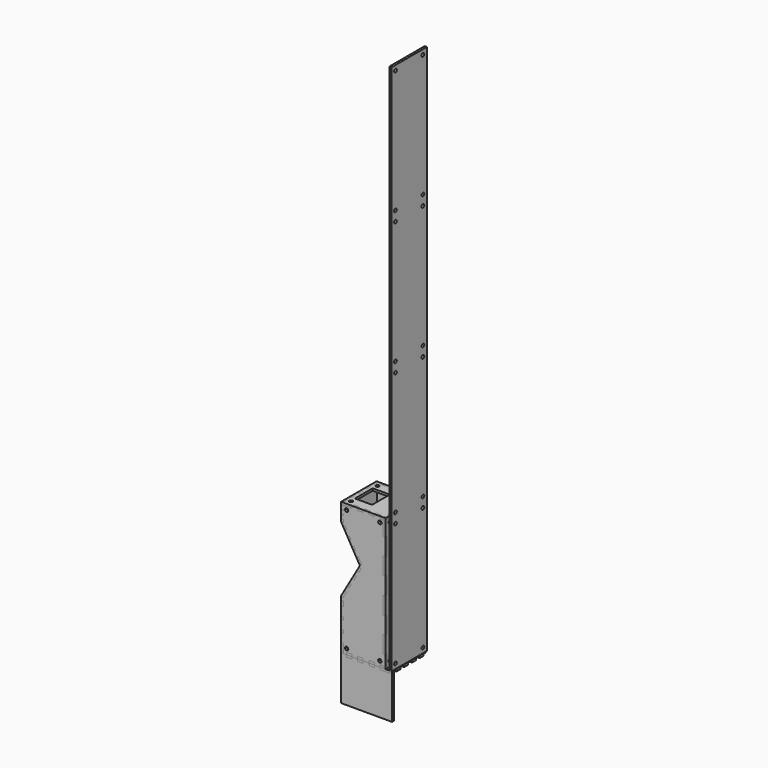
from build123d import *

# Parameters (mm, degrees)
F5_W      = 6
F5_H      = 4
F5_W_2    = 10
F5_W_3    = 4
F5_H_2    = 4.9052353799
F5_H_3    = 8.75
F5_R      = 3
F5_W_4    = 31
F5_H_4    = 40
F5_H_5    = 5.8447646201
F25_DEPTH = 4
F7_R      = 3
F7_W      = 4
F7_H      = 30
F7_H_2    = 31.25
F7_H_3    = 22.5
F26_DEPTH = 4
F3_R      = 3
F27_DEPTH = 4
F9_W      = 6
F9_H      = 4
F9_W_2    = 10
F9_R      = 3
F9_W_3    = 4
F9_H_2    = 14.5947646201
F9_H_3    = 8.75
F9_H_4    = 4.9052353799
F28_DEPTH = 4
F11_R     = 3
F29_DEPTH = 4
F30_DEPTH = 4
F31_DEPTH = 4
F32_DEPTH = 4
F33_DEPTH = 4
F34_DEPTH = 4
F35_DEPTH = 4
F36_DEPTH = 4
F37_DEPTH = 4
F38_DEPTH = 4
F19_R     = 25
F39_DEPTH = 4
F40_DEPTH = 4
F22_W     = 80
F22_H     = 240
F22_R     = 3
F41_DEPTH = 4
F24_R     = 3
F24_W     = 31
F24_H     = 40
F42_DEPTH = 4
F43_DEPTH = 4
F23_W     = 6
F23_H     = 4
F23_W_2   = 4
F23_H_2   = 8.75
F23_W_3   = 10
F23_H_3   = 4.9052353799
F44_DEPTH = 4
F23_H_4   = 5.8447646201
F45_DEPTH = 4


# Not quite as in the source:
# - a feature names something its author has since deleted; it is built from what else it names


with BuildPart() as f25:
    # F5 (on line) → F25 (new body)
    with BuildSketch(Plane.XY.offset(240)):
        with Locations((-73, 78)):
            Rectangle(F5_W, F5_H)
        with Locations((-55, 78)):
            Rectangle(F5_W_2, F5_H)
        with Locations((-35, 78)):
            Rectangle(F5_W_2, F5_H)
        with Locations((-15, 78)):
            Rectangle(F5_W_2, F5_H)
        with Locations((-2, 78)):
            Rectangle(F5_W_3, F5_H)
        with Locations((-2, 73.54738231)):
            Rectangle(F5_W_3, F5_H_2)
        with Locations((-2, 57.9697646201)):
            Rectangle(F5_W_3, F5_H_3)
        with Locations((-2, 40.4697646201)):
            Rectangle(F5_W_3, F5_H_3)
        with Locations((-2, 22.9697646201)):
            Rectangle(F5_W_3, F5_H_3)
        with Locations((-25, 2)):
            Rectangle(F5_W_2, F5_H)
        with Locations((-45, 2)):
            Rectangle(F5_W_2, F5_H)
        with Locations((-65, 2)):
            Rectangle(F5_W_2, F5_H)
        with Locations((-78, 66.7197646201)):
            Rectangle(F5_W_3, F5_H_3)
        with Locations((-78, 49.2197646201)):
            Rectangle(F5_W_3, F5_H_3)
        with Locations((-78, 31.7197646201)):
            Rectangle(F5_W_3, F5_H_3)
        with Locations((-78, 14.2197646201)):
            Rectangle(F5_W_3, F5_H_3)
        Polygon((-76, 9.8447646201), (-76, 4), (-70, 4), (-60, 4), (-50, 4), (-40, 4), (-30, 4), (-20, 4), (-10, 4), (-4, 4), (-4, 9.8447646201), (-4, 18.5947646201), (-4, 27.3447646201), (-4, 36.0947646201), (-4, 44.8447646201), (-4, 53.5947646201), (-4, 62.3447646201), (-4, 71.0947646201), (-4, 76), (-10, 76), (-20, 76), (-30, 76), (-40, 76), (-50, 76), (-60, 76), (-70, 76), (-76, 76), (-76, 71.0947646201), (-76, 62.3447646201), (-76, 53.5947646201), (-76, 44.8447646201), (-76, 36.0947646201), (-76, 27.3447646201), (-76, 18.5947646201), align=None)
        with Locations((-70, 10)):
            Circle(F5_R, mode=Mode.SUBTRACT)
        with Locations((-55.5, 40)):
            Rectangle(F5_W_4, F5_H_4, mode=Mode.SUBTRACT)
        with Locations((-70, 70)):
            Circle(F5_R, mode=Mode.SUBTRACT)
        with Locations((-10, 40)):
            Circle(F5_R, mode=Mode.SUBTRACT)
        with Locations((-2, 6.92238231)):
            Rectangle(F5_W_3, F5_H_5)
        with Locations((-7, 2)):
            Rectangle(F5_W, F5_H)
        with Locations((-78, 2)):
            Rectangle(F5_W_3, F5_H)
        with Locations((-73, 2)):
            Rectangle(F5_W, F5_H)
    extrude(amount=-F25_DEPTH)


with BuildPart() as f26:
    # F7 (on line) → F26 (new body)
    with BuildSketch(Plane.YZ):
        Polygon((4, 22.5), (4, 0), (76, 0), (76, 22.5), (76, 53.75), (76, 85), (76, 116.25), (76, 147.5), (76, 178.75), (76, 210), (76, 240), (4, 240), (4, 210), (4, 178.75), (4, 147.5), (4, 116.25), (4, 85), (4, 53.75), align=None)
        with Locations((10, 10)):
            Circle(F7_R, mode=Mode.SUBTRACT)
        with Locations((70, 10)):
            Circle(F7_R, mode=Mode.SUBTRACT)
        with Locations((10, 230)):
            Circle(F7_R, mode=Mode.SUBTRACT)
        with Locations((70, 230)):
            Circle(F7_R, mode=Mode.SUBTRACT)
        with Locations((2, 225)):
            Rectangle(F7_W, F7_H)
        with Locations((2, 163.125)):
            Rectangle(F7_W, F7_H_2)
        with Locations((2, 100.625)):
            Rectangle(F7_W, F7_H_2)
        with Locations((2, 38.125)):
            Rectangle(F7_W, F7_H_2)
        with Locations((78, 11.25)):
            Rectangle(F7_W, F7_H_3)
        with Locations((78, 69.375)):
            Rectangle(F7_W, F7_H_2)
        with Locations((78, 131.875)):
            Rectangle(F7_W, F7_H_2)
        with Locations((78, 194.375)):
            Rectangle(F7_W, F7_H_2)
    extrude(amount=-F26_DEPTH)


with BuildPart() as f27:
    # F3 (on Front) → F27 (new body)
    with BuildSketch(Plane.XZ):
        Polygon((0, 240), (-80, 240), (-80, 208.334591186), (-46, 149.4448637287), (-80, 90.5551362713), (-80, 0), (0, 0), align=None)
        with Locations((-70, 10)):
            Circle(F3_R, mode=Mode.SUBTRACT)
        with Locations((-10, 10)):
            Circle(F3_R, mode=Mode.SUBTRACT)
        with Locations((-70, 230)):
            Circle(F3_R, mode=Mode.SUBTRACT)
        with Locations((-10, 230)):
            Circle(F3_R, mode=Mode.SUBTRACT)
    extrude(amount=-F27_DEPTH)


with BuildPart() as f28:
    # F9 (on line) → F28 (new body)
    with BuildSketch(Plane.XY):
        with Locations((-7, 2)):
            Rectangle(F9_W, F9_H)
        with Locations((-25, 2)):
            Rectangle(F9_W_2, F9_H)
        with Locations((-45, 2)):
            Rectangle(F9_W_2, F9_H)
        with Locations((-65, 2)):
            Rectangle(F9_W_2, F9_H)
        Polygon((-76, 18.5947646201), (-76, 4), (-70, 4), (-60, 4), (-50, 4), (-40, 4), (-30, 4), (-20, 4), (-10, 4), (-4, 4), (-4, 18.5947646201), (-4, 27.3447646201), (-4, 36.0947646201), (-4, 44.8447646201), (-4, 53.5947646201), (-4, 62.3447646201), (-4, 71.0947646201), (-4, 76), (-10, 76), (-20, 76), (-30, 76), (-40, 76), (-50, 76), (-60, 76), (-70, 76), (-76, 76), (-76, 71.0947646201), (-76, 62.3447646201), (-76, 53.5947646201), (-76, 44.8447646201), (-76, 36.0947646201), (-76, 27.3447646201), align=None)
        with Locations((-70, 10)):
            Circle(F9_R, mode=Mode.SUBTRACT)
        with BuildLine():
            ThreePointArc((-65, 32), (-68, 29), (-71, 32))
            ThreePointArc((-71, 32), (-68, 35), (-65, 32))
        make_face(mode=Mode.SUBTRACT)
        with Locations((-60, 36)):
            Circle(F9_R, mode=Mode.SUBTRACT)
        with BuildLine():
            ThreePointArc((-65, 40), (-68, 37), (-71, 40))
            ThreePointArc((-71, 40), (-68, 43), (-65, 40))
        make_face(mode=Mode.SUBTRACT)
        with BuildLine():
            ThreePointArc((-65, 48), (-68, 45), (-71, 48))
            ThreePointArc((-71, 48), (-68, 51), (-65, 48))
        make_face(mode=Mode.SUBTRACT)
        with Locations((-60, 44)):
            Circle(F9_R, mode=Mode.SUBTRACT)
        with Locations((-52, 40)):
            Circle(F9_R, mode=Mode.SUBTRACT)
        with Locations((-70, 70)):
            Circle(F9_R, mode=Mode.SUBTRACT)
        with BuildLine():
            ThreePointArc((-9, 42.8284271247), (-7.5505102572, 41.7320508076), (-7, 40))
            ThreePointArc((-7, 40), (-12.4494897428, 38.2679491924), (-9, 42.8284271247))
        make_face(mode=Mode.SUBTRACT)
        with Locations((-78, 11.29738231)):
            Rectangle(F9_W_3, F9_H_2)
        with Locations((-78, 31.7197646201)):
            Rectangle(F9_W_3, F9_H_3)
        with Locations((-2, 22.9697646201)):
            Rectangle(F9_W_3, F9_H_3)
        with Locations((-2, 40.4697646201)):
            Rectangle(F9_W_3, F9_H_3)
        with Locations((-2, 57.9697646201)):
            Rectangle(F9_W_3, F9_H_3)
        with Locations((-2, 73.54738231)):
            Rectangle(F9_W_3, F9_H_4)
        with Locations((-2, 78)):
            Rectangle(F9_W_3, F9_H)
        with Locations((-15, 78)):
            Rectangle(F9_W_2, F9_H)
        with Locations((-35, 78)):
            Rectangle(F9_W_2, F9_H)
        with Locations((-55, 78)):
            Rectangle(F9_W_2, F9_H)
        with Locations((-73, 78)):
            Rectangle(F9_W, F9_H)
        with Locations((-78, 66.7197646201)):
            Rectangle(F9_W_3, F9_H_3)
        with Locations((-78, 49.2197646201)):
            Rectangle(F9_W_3, F9_H_3)
        with Locations((-78, 2)):
            Rectangle(F9_W_3, F9_H)
    extrude(amount=F28_DEPTH)


with BuildPart() as f29:
    # F11 (on line) → F29 (new body)
    with BuildSketch(Plane(origin=(0, 80, 0), x_dir=(-1, 0, 0), z_dir=(0, 1, 0))):
        Polygon((46, 149.4448637287), (80, 208.334591186), (80, 240), (0, 240), (0, 0), (80, 0), (80, 90.5551362713), align=None)
        with Locations((10, 10)):
            Circle(F11_R, mode=Mode.SUBTRACT)
        with Locations((70, 10)):
            Circle(F11_R, mode=Mode.SUBTRACT)
        with Locations((10, 230)):
            Circle(F11_R, mode=Mode.SUBTRACT)
        with Locations((70, 230)):
            Circle(F11_R, mode=Mode.SUBTRACT)
    extrude(amount=-F29_DEPTH)


with BuildPart() as f30:
    # F13 (on line) → F30 (new body)
    with BuildSketch(Plane.YZ.offset(-80)):
        Polygon((0, 213.0509433895), (0, 208.334591186), (80, 208.334591186), (80, 213.0509433895), (76, 213.0509433895), (76, 216.2509433895), (76, 219.4509433895), (80, 219.4509433895), (80, 220.967295593), (76, 220.967295593), (76, 224.167295593), (76, 227.367295593), (80, 227.367295593), (80, 228.8836477965), (76, 228.8836477965), (76, 232.0836477965), (76, 235.2836477965), (80, 235.2836477965), (80, 240), (0, 240), (0, 235.2836477965), (4, 235.2836477965), (4, 232.0836477965), (4, 228.8836477965), (0, 228.8836477965), (0, 227.367295593), (4, 227.367295593), (4, 224.167295593), (4, 220.967295593), (0, 220.967295593), (0, 219.4509433895), (4, 219.4509433895), (4, 216.2509433895), (4, 213.0509433895), align=None)
    extrude(amount=F30_DEPTH)


with BuildPart() as f31:
    # F15 (on line) → F31 (new body)
    with BuildSketch(Plane.YZ.offset(-80)):
        Polygon((76.0003124634, 53.2275720415), (80, 53.2775681357), (80, 58.4163522035), (76.0003124634, 58.4163522035), (76.0003124634, 66.4163522035), (76.0003124634, 74.4163522035), (80, 74.4163522035), (80, 83.5551362713), (76.0003124634, 83.5551362713), (76.0003124634, 88.5551362713), (3.9996875366, 88.5551362713), (3.9996875366, 83.5551362713), (0, 83.5551362713), (0, 74.4163522035), (3.9996875366, 74.4163522035), (3.9996875366, 66.4163522035), (3.9996875366, 58.4163522035), (0, 58.4163522035), (0, 53.2775681357), (3.9996875366, 53.2275720415), (3.9996875366, 45.2275720415), (3.7997187817, 37.2300716509), (0, 37.2775681357), (0, 32.1346775562), (3.6700195432, 32.0429127293), (3.4700507883, 24.0454123388), (3.2700820334, 16.0479119482), (0, 16.1296767748), (0, 0), (80, 0), (80, 16.1296767748), (76.7299179666, 16.0479119482), (76.5299492117, 24.0454123388), (76.3299804568, 32.0429127293), (80, 32.1346775562), (80, 37.2775681357), (76.2002812183, 37.2300716509), (76.0003124634, 45.2275720415), align=None)
    extrude(amount=F31_DEPTH)


with BuildPart() as f32_tool:
    # F5 (on line) → F32 (new body)
    with BuildSketch(Plane.XY.offset(240)):
        with Locations((-2, 22.9697646201)):
            Rectangle(F5_W_3, F5_H_3)
        with Locations((-2, 40.4697646201)):
            Rectangle(F5_W_3, F5_H_3)
        with Locations((-2, 57.9697646201)):
            Rectangle(F5_W_3, F5_H_3)
        with Locations((-2, 73.54738231)):
            Rectangle(F5_W_3, F5_H_2)
        with Locations((-2, 78)):
            Rectangle(F5_W_3, F5_H)
        with Locations((-15, 78)):
            Rectangle(F5_W_2, F5_H)
        with Locations((-35, 78)):
            Rectangle(F5_W_2, F5_H)
        with Locations((-55, 78)):
            Rectangle(F5_W_2, F5_H)
        with Locations((-73, 78)):
            Rectangle(F5_W, F5_H)
        with Locations((-78, 66.7197646201)):
            Rectangle(F5_W_3, F5_H_3)
        with Locations((-78, 49.2197646201)):
            Rectangle(F5_W_3, F5_H_3)
        with Locations((-78, 31.7197646201)):
            Rectangle(F5_W_3, F5_H_3)
        with Locations((-78, 14.2197646201)):
            Rectangle(F5_W_3, F5_H_3)
        with Locations((-78, 2)):
            Rectangle(F5_W_3, F5_H)
        with Locations((-65, 2)):
            Rectangle(F5_W_2, F5_H)
        with Locations((-45, 2)):
            Rectangle(F5_W_2, F5_H)
        with Locations((-25, 2)):
            Rectangle(F5_W_2, F5_H)
        with Locations((-7, 2)):
            Rectangle(F5_W, F5_H)
        with Locations((-73, 2)):
            Rectangle(F5_W, F5_H)
        with Locations((-2, 6.92238231)):
            Rectangle(F5_W_3, F5_H_5)
    extrude(amount=-F32_DEPTH)


with BuildPart() as f26_1:
    add(f26.part)

    # F32: cut by f32_tool
    add(f32_tool.part, mode=Mode.SUBTRACT)


with BuildPart() as f27_1:
    add(f27.part)

    # F32: cut by f32_tool
    add(f32_tool.part, mode=Mode.SUBTRACT)


with BuildPart() as f29_1:
    add(f29.part)

    # F32: cut by f32_tool
    add(f32_tool.part, mode=Mode.SUBTRACT)


with BuildPart() as f30_1:
    add(f30.part)

    # F32: cut by f32_tool
    add(f32_tool.part, mode=Mode.SUBTRACT)


with BuildPart() as f33_tool:
    # F7 (on line) → F33 (new body)
    with BuildSketch(Plane.YZ):
        with Locations((2, 225)):
            Rectangle(F7_W, F7_H)
        with Locations((78, 194.375)):
            Rectangle(F7_W, F7_H_2)
        with Locations((2, 163.125)):
            Rectangle(F7_W, F7_H_2)
        with Locations((78, 131.875)):
            Rectangle(F7_W, F7_H_2)
        with Locations((2, 100.625)):
            Rectangle(F7_W, F7_H_2)
        with Locations((78, 69.375)):
            Rectangle(F7_W, F7_H_2)
        with Locations((2, 38.125)):
            Rectangle(F7_W, F7_H_2)
        with Locations((78, 11.25)):
            Rectangle(F7_W, F7_H_3)
    extrude(amount=-F33_DEPTH)


with BuildPart() as f27_2:
    add(f27_1.part)

    # F33: cut by f33_tool
    add(f33_tool.part, mode=Mode.SUBTRACT)


with BuildPart() as f29_2:
    add(f29_1.part)

    # F33: cut by f33_tool
    add(f33_tool.part, mode=Mode.SUBTRACT)


with BuildPart() as f34_tool:
    # F13 (on line) → F34 (new body)
    with BuildSketch(Plane.YZ.offset(-80)):
        Polygon((0, 213.0509433895), (0, 208.334591186), (80, 208.334591186), (80, 213.0509433895), (76, 213.0509433895), (76, 216.2509433895), (76, 219.4509433895), (80, 219.4509433895), (80, 220.967295593), (76, 220.967295593), (76, 224.167295593), (76, 227.367295593), (80, 227.367295593), (80, 228.8836477965), (76, 228.8836477965), (76, 232.0836477965), (76, 235.2836477965), (80, 235.2836477965), (80, 240), (0, 240), (0, 235.2836477965), (4, 235.2836477965), (4, 232.0836477965), (4, 228.8836477965), (0, 228.8836477965), (0, 227.367295593), (4, 227.367295593), (4, 224.167295593), (4, 220.967295593), (0, 220.967295593), (0, 219.4509433895), (4, 219.4509433895), (4, 216.2509433895), (4, 213.0509433895), align=None)
    extrude(amount=F34_DEPTH)


with BuildPart() as f27_3:
    add(f27_2.part)

    # F34: cut by f34_tool
    add(f34_tool.part, mode=Mode.SUBTRACT)


with BuildPart() as f29_3:
    add(f29_2.part)

    # F34: cut by f34_tool
    add(f34_tool.part, mode=Mode.SUBTRACT)


with BuildPart() as f35_tool:
    # F15 (on line) → F35 (new body)
    with BuildSketch(Plane.YZ.offset(-80)):
        Polygon((76.0003124634, 53.2275720415), (80, 53.2775681357), (80, 58.4163522035), (76.0003124634, 58.4163522035), (76.0003124634, 66.4163522035), (76.0003124634, 74.4163522035), (80, 74.4163522035), (80, 83.5551362713), (76.0003124634, 83.5551362713), (76.0003124634, 88.5551362713), (3.9996875366, 88.5551362713), (3.9996875366, 83.5551362713), (0, 83.5551362713), (0, 74.4163522035), (3.9996875366, 74.4163522035), (3.9996875366, 66.4163522035), (3.9996875366, 58.4163522035), (0, 58.4163522035), (0, 53.2775681357), (3.9996875366, 53.2275720415), (3.9996875366, 45.2275720415), (3.7997187817, 37.2300716509), (0, 37.2775681357), (0, 32.1346775562), (3.6700195432, 32.0429127293), (3.4700507883, 24.0454123388), (3.2700820334, 16.0479119482), (0, 16.1296767748), (0, 0), (80, 0), (80, 16.1296767748), (76.7299179666, 16.0479119482), (76.5299492117, 24.0454123388), (76.3299804568, 32.0429127293), (80, 32.1346775562), (80, 37.2775681357), (76.2002812183, 37.2300716509), (76.0003124634, 45.2275720415), align=None)
    extrude(amount=F35_DEPTH)


with BuildPart() as f27_4:
    add(f27_3.part)

    # F35: cut by f35_tool
    add(f35_tool.part, mode=Mode.SUBTRACT)


with BuildPart() as f29_4:
    add(f29_3.part)

    # F35: cut by f35_tool
    add(f35_tool.part, mode=Mode.SUBTRACT)


with BuildPart() as f36_tool:
    # F9 (on line) → F36 (new body)
    with BuildSketch(Plane.XY):
        with Locations((-73, 78)):
            Rectangle(F9_W, F9_H)
        with Locations((-78, 66.7197646201)):
            Rectangle(F9_W_3, F9_H_3)
        with Locations((-55, 78)):
            Rectangle(F9_W_2, F9_H)
        with Locations((-35, 78)):
            Rectangle(F9_W_2, F9_H)
        with Locations((-15, 78)):
            Rectangle(F9_W_2, F9_H)
        with Locations((-2, 78)):
            Rectangle(F9_W_3, F9_H)
        with Locations((-2, 73.54738231)):
            Rectangle(F9_W_3, F9_H_4)
        with Locations((-2, 57.9697646201)):
            Rectangle(F9_W_3, F9_H_3)
        with Locations((-2, 40.4697646201)):
            Rectangle(F9_W_3, F9_H_3)
        with Locations((-2, 22.9697646201)):
            Rectangle(F9_W_3, F9_H_3)
        with Locations((-7, 2)):
            Rectangle(F9_W, F9_H)
        with Locations((-25, 2)):
            Rectangle(F9_W_2, F9_H)
        with Locations((-45, 2)):
            Rectangle(F9_W_2, F9_H)
        with Locations((-65, 2)):
            Rectangle(F9_W_2, F9_H)
        with Locations((-78, 2)):
            Rectangle(F9_W_3, F9_H)
        with Locations((-78, 11.29738231)):
            Rectangle(F9_W_3, F9_H_2)
        with Locations((-78, 31.7197646201)):
            Rectangle(F9_W_3, F9_H_3)
        with Locations((-78, 49.2197646201)):
            Rectangle(F9_W_3, F9_H_3)
    extrude(amount=F36_DEPTH)


with BuildPart() as f26_2:
    add(f26_1.part)

    # F36: cut by f36_tool
    add(f36_tool.part, mode=Mode.SUBTRACT)


with BuildPart() as f27_5:
    add(f27_4.part)

    # F36: cut by f36_tool
    add(f36_tool.part, mode=Mode.SUBTRACT)


with BuildPart() as f29_5:
    add(f29_4.part)

    # F36: cut by f36_tool
    add(f36_tool.part, mode=Mode.SUBTRACT)


with BuildPart() as f31_1:
    add(f31.part)

    # F36: cut by f36_tool
    add(f36_tool.part, mode=Mode.SUBTRACT)


with BuildPart() as f37:
    # F17 (on line) → F37 (new body)
    with BuildSketch(Plane(origin=(30.2115242271, 0, 17.4426316451), x_dir=(0, 1, 0), z_dir=(0.8660254038, 0, 0.5))):
        Polygon((0, 165.4230484541), (0, 153.5777489925), (80, 153.5777489925), (80, 165.4230484541), (76, 165.4230484541), (76, 170.4230484541), (76, 175.4230484541), (80, 175.4230484541), (80, 181.4230484541), (76, 181.4230484541), (76, 186.4230484541), (76, 191.4230484541), (80, 191.4230484541), (80, 197.4230484541), (76, 197.4230484541), (76, 202.4230484541), (76, 207.4230484541), (80, 207.4230484541), (80, 213.4230484541), (76, 213.4230484541), (76, 218.4230484541), (4, 218.4230484541), (4, 213.4230484541), (0, 213.4230484541), (0, 207.4230484541), (4, 207.4230484541), (4, 202.4230484541), (4, 197.4230484541), (0, 197.4230484541), (0, 191.4230484541), (4, 191.4230484541), (4, 186.4230484541), (4, 181.4230484541), (0, 181.4230484541), (0, 175.4230484541), (4, 175.4230484541), (4, 170.4230484541), (4, 165.4230484541), align=None)
    extrude(amount=F37_DEPTH)


with BuildPart() as f38_tool:
    # F17 (on line) → F38 (new body)
    with BuildSketch(Plane(origin=(30.2115242271, 0, 17.4426316451), x_dir=(0, 1, 0), z_dir=(0.8660254038, 0, 0.5))):
        Polygon((0, 165.4230484541), (0, 153.5777489925), (80, 153.5777489925), (80, 165.4230484541), (76, 165.4230484541), (76, 170.4230484541), (76, 175.4230484541), (80, 175.4230484541), (80, 181.4230484541), (76, 181.4230484541), (76, 186.4230484541), (76, 191.4230484541), (80, 191.4230484541), (80, 197.4230484541), (76, 197.4230484541), (76, 202.4230484541), (76, 207.4230484541), (80, 207.4230484541), (80, 213.4230484541), (76, 213.4230484541), (76, 218.4230484541), (4, 218.4230484541), (4, 213.4230484541), (0, 213.4230484541), (0, 207.4230484541), (4, 207.4230484541), (4, 202.4230484541), (4, 197.4230484541), (0, 197.4230484541), (0, 191.4230484541), (4, 191.4230484541), (4, 186.4230484541), (4, 181.4230484541), (0, 181.4230484541), (0, 175.4230484541), (4, 175.4230484541), (4, 170.4230484541), (4, 165.4230484541), align=None)
    extrude(amount=F38_DEPTH)


with BuildPart() as f27_6:
    add(f27_5.part)

    # F38: cut by f38_tool
    add(f38_tool.part, mode=Mode.SUBTRACT)


with BuildPart() as f29_6:
    add(f29_5.part)

    # F38: cut by f38_tool
    add(f38_tool.part, mode=Mode.SUBTRACT)


with BuildPart() as f39:
    # F19 (on line) → F39 (new body)
    with BuildSketch(Plane(origin=(-99.2115242271, 0, 57.2798002192), x_dir=(0, 1, 0), z_dir=(0.8660254038, 0, -0.5))):
        Polygon((0, 51.0003987233), (0, 38.4230484541), (80, 38.4230484541), (80, 51.0003987233), (76, 51.0003987233), (76, 56.0003987233), (76, 61.0003987233), (80, 61.0003987233), (80, 68.5777489925), (76, 68.5777489925), (76, 73.5777489925), (76, 78.5777489925), (80, 78.5777489925), (80, 86.1550992617), (76, 86.1550992617), (76, 91.1550992617), (76, 96.1550992617), (80, 96.1550992617), (80, 103.7324495309), (76, 103.7324495309), (76, 108.7324495309), (4, 108.7324495309), (4, 103.7324495309), (0, 103.7324495309), (0, 96.1550992617), (4, 96.1550992617), (4, 91.1550992617), (4, 86.1550992617), (0, 86.1550992617), (0, 78.5777489925), (4, 78.5777489925), (4, 73.5777489925), (4, 68.5777489925), (0, 68.5777489925), (0, 61.0003987233), (4, 61.0003987233), (4, 56.0003987233), (4, 51.0003987233), align=None)
        with Locations((40, 73.5777489925)):
            Circle(F19_R, mode=Mode.SUBTRACT)
    extrude(amount=F39_DEPTH)


with BuildPart() as f40_tool:
    # F19 (on line) → F40 (new body)
    with BuildSketch(Plane(origin=(-99.2115242271, 0, 57.2798002192), x_dir=(0, 1, 0), z_dir=(0.8660254038, 0, -0.5))):
        Polygon((0, 51.0003987233), (0, 38.4230484541), (80, 38.4230484541), (80, 51.0003987233), (76, 51.0003987233), (76, 56.0003987233), (76, 61.0003987233), (80, 61.0003987233), (80, 68.5777489925), (76, 68.5777489925), (76, 73.5777489925), (76, 78.5777489925), (80, 78.5777489925), (80, 86.1550992617), (76, 86.1550992617), (76, 91.1550992617), (76, 96.1550992617), (80, 96.1550992617), (80, 103.7324495309), (76, 103.7324495309), (76, 108.7324495309), (4, 108.7324495309), (4, 103.7324495309), (0, 103.7324495309), (0, 96.1550992617), (4, 96.1550992617), (4, 91.1550992617), (4, 86.1550992617), (0, 86.1550992617), (0, 78.5777489925), (4, 78.5777489925), (4, 73.5777489925), (4, 68.5777489925), (0, 68.5777489925), (0, 61.0003987233), (4, 61.0003987233), (4, 56.0003987233), (4, 51.0003987233), align=None)
        with Locations((40, 73.5777489925)):
            Circle(F19_R, mode=Mode.SUBTRACT)
    extrude(amount=F40_DEPTH)


with BuildPart() as f27_7:
    add(f27_6.part)

    # F40: cut by f40_tool
    add(f40_tool.part, mode=Mode.SUBTRACT)


with BuildPart() as f29_7:
    add(f29_6.part)

    # F40: cut by f40_tool
    add(f40_tool.part, mode=Mode.SUBTRACT)


with BuildPart() as f41:
    # F22 (on offset) → F41 (new body)
    with BuildSketch(Plane.YZ.offset(11)):
        with Locations((40, 120)):
            Rectangle(F22_W, F22_H)
        with Locations((9, 9)):
            Circle(F22_R, mode=Mode.SUBTRACT)
        with Locations((9, 231)):
            Circle(F22_R, mode=Mode.SUBTRACT)
        with Locations((71, 9)):
            Circle(F22_R, mode=Mode.SUBTRACT)
        with Locations((71, 231)):
            Circle(F22_R, mode=Mode.SUBTRACT)
        with Locations((40, 360)):
            Rectangle(F22_W, F22_H)
        with Locations((9, 249)):
            Circle(F22_R, mode=Mode.SUBTRACT)
        with Locations((9, 471)):
            Circle(F22_R, mode=Mode.SUBTRACT)
        with Locations((71, 249)):
            Circle(F22_R, mode=Mode.SUBTRACT)
        with Locations((71, 471)):
            Circle(F22_R, mode=Mode.SUBTRACT)
        with Locations((40, 600)):
            Rectangle(F22_W, F22_H)
        with Locations((9, 489)):
            Circle(F22_R, mode=Mode.SUBTRACT)
        with Locations((9, 711)):
            Circle(F22_R, mode=Mode.SUBTRACT)
        with Locations((71, 489)):
            Circle(F22_R, mode=Mode.SUBTRACT)
        with Locations((71, 711)):
            Circle(F22_R, mode=Mode.SUBTRACT)
        with Locations((40, 840)):
            Rectangle(F22_W, F22_H)
        with Locations((9, 729)):
            Circle(F22_R, mode=Mode.SUBTRACT)
        with Locations((9, 951)):
            Circle(F22_R, mode=Mode.SUBTRACT)
        with Locations((71, 729)):
            Circle(F22_R, mode=Mode.SUBTRACT)
        with Locations((71, 951)):
            Circle(F22_R, mode=Mode.SUBTRACT)
    extrude(amount=-F41_DEPTH)


with BuildPart() as f42:
    # F24 (on line) → F42 (new body)
    with BuildSketch(Plane.XY):
        Polygon((0, 80), (-80, 80), (-80, 0), (0, 0), (12, 0), (12, 80), align=None)
        with Locations((-70, 10)):
            Circle(F24_R, mode=Mode.SUBTRACT)
        with Locations((-55.5, 40)):
            Rectangle(F24_W, F24_H, mode=Mode.SUBTRACT)
        with Locations((-70, 70)):
            Circle(F24_R, mode=Mode.SUBTRACT)
        with Locations((-10, 40)):
            Circle(F24_R, mode=Mode.SUBTRACT)
    extrude(amount=-F42_DEPTH)

    # F23 (on line) → F44 (cut)
    with BuildSketch(Plane.XY):
        with Locations((-73, 78)):
            Rectangle(F23_W, F23_H)
        with Locations((-78, 66.7197646201)):
            Rectangle(F23_W_2, F23_H_2)
        with Locations((-78, 49.2197646201)):
            Rectangle(F23_W_2, F23_H_2)
        with Locations((-78, 31.7197646201)):
            Rectangle(F23_W_2, F23_H_2)
        with Locations((-78, 14.2197646201)):
            Rectangle(F23_W_2, F23_H_2)
        with Locations((-78, 2)):
            Rectangle(F23_W_2, F23_H)
        with Locations((-73, 2)):
            Rectangle(F23_W, F23_H)
        with Locations((-55, 2)):
            Rectangle(F23_W_3, F23_H)
        Polygon((-30, 4), (-31, 4), (-40, 4), (-40, 0), (-30, 0), align=None)
        with Locations((-15, 2)):
            Rectangle(F23_W_3, F23_H)
        with Locations((10, 2)):
            Rectangle(F23_W_2, F23_H)
        Polygon((8, 9.8447646201), (8, 4), (12, 4), (12, 9.6828316604), align=None)
        with Locations((10, 22.9697646201)):
            Rectangle(F23_W_2, F23_H_2)
        with Locations((10, 40.4697646201)):
            Rectangle(F23_W_2, F23_H_2)
        with Locations((10, 57.9697646201)):
            Rectangle(F23_W_2, F23_H_2)
        with Locations((10, 73.54738231)):
            Rectangle(F23_W_2, F23_H_3)
        with Locations((10, 78)):
            Rectangle(F23_W_2, F23_H)
        with Locations((-15, 78)):
            Rectangle(F23_W_3, F23_H)
        Polygon((-30, 80), (-40, 80), (-40, 76), (-31, 76), (-30, 76), align=None)
        with Locations((-55, 78)):
            Rectangle(F23_W_3, F23_H)
    extrude(amount=-F44_DEPTH, mode=Mode.SUBTRACT)


with BuildPart() as f43:
    # F3 (on Front) → F43 (new body)
    with BuildSketch(Plane.XZ):
        Polygon((12, 0), (0, 0), (-80, 0), (-80, -80), (0, -80), (12, -80), align=None)
    extrude(amount=-F43_DEPTH)

    # F23 (on line) → F45 (cut)
    with BuildSketch(Plane.XY):
        with Locations((-65, 2)):
            Rectangle(F23_W_3, F23_H)
        with Locations((-45, 2)):
            Rectangle(F23_W_3, F23_H)
        Polygon((-20, 4), (-27, 4), (-30, 4), (-30, 0), (-20, 0), align=None)
        Polygon((0, 4), (-10, 4), (-10, 0), (0, 0), (8, 0), (8, 4), align=None)
        Polygon((8, 18.5947646201), (8, 9.8447646201), (12, 9.6828316604), (12, 18.5947646201), align=None)
        with Locations((10, 31.7197646201)):
            Rectangle(F23_W_2, F23_H_2)
        with Locations((10, 49.2197646201)):
            Rectangle(F23_W_2, F23_H_2)
        with Locations((10, 66.7197646201)):
            Rectangle(F23_W_2, F23_H_2)
        Polygon((0, 80), (-10, 80), (-10, 76), (0, 76), (8, 76), (8, 80), align=None)
        Polygon((-20, 80), (-30, 80), (-30, 76), (-27, 76), (-20, 76), align=None)
        with Locations((-45, 78)):
            Rectangle(F23_W_3, F23_H)
        with Locations((-65, 78)):
            Rectangle(F23_W_3, F23_H)
        with Locations((-78, 73.54738231)):
            Rectangle(F23_W_2, F23_H_3)
        with Locations((-78, 57.9697646201)):
            Rectangle(F23_W_2, F23_H_2)
        with Locations((-78, 40.4697646201)):
            Rectangle(F23_W_2, F23_H_2)
        with Locations((-78, 22.9697646201)):
            Rectangle(F23_W_2, F23_H_2)
        with Locations((-78, 6.92238231)):
            Rectangle(F23_W_2, F23_H_4)
    extrude(amount=-F45_DEPTH, mode=Mode.SUBTRACT)


solid = Compound([f25.part, f28.part, f30_1.part, f26_2.part, f31_1.part, f37.part, f39.part, f27_7.part, f29_7.part, f41.part, f42.part, f43.part])
